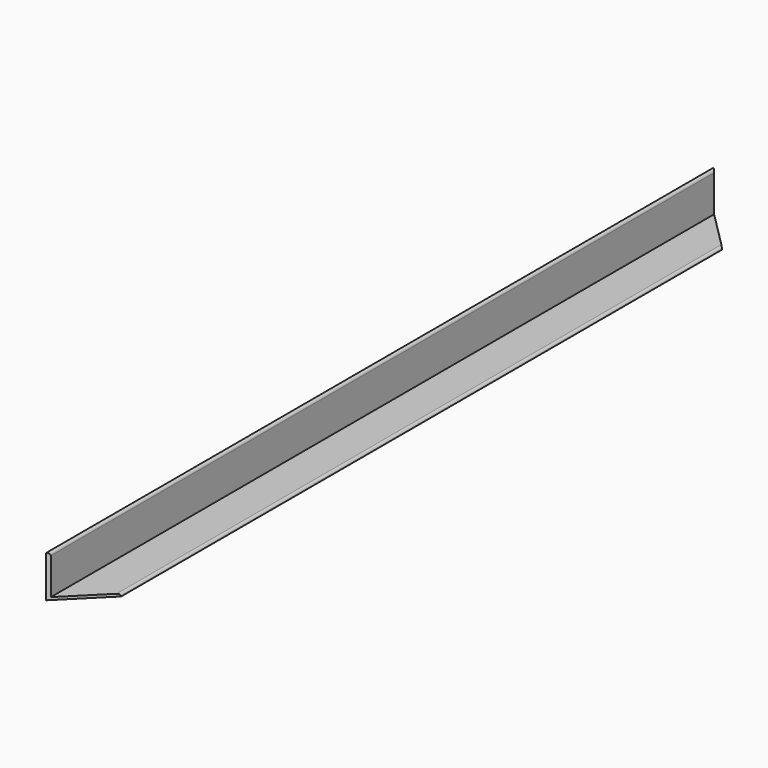
from build123d import *

# Parameters (mm, degrees)
F1_DEPTH = 508
F3_DEPTH = 50.8


# Not quite as in the source:
# - a pattern or mirror of a feature is missing from the dataset's text; its kind, count and spacing are read off the source's solid


with BuildPart() as f1:
    # F0 (on Front) → F1 (new body, symmetric)
    with BuildSketch(Plane.XZ):
        with BuildLine():
            ThreePointArc((-920.7500404358, 47.625), (-921.6799764055, 49.8700640303), (-923.9250404358, 50.8))
            Line((-923.9250404358, 50.8), (-923.9250404358, 0))
            Line((-923.9250404358, 0), (-873.1250404358, 0))
            ThreePointArc((-873.1250404358, 0), (-874.0549764055, 2.2450640303), (-876.3000404358, 3.175))
            Line((-876.3000404358, 3.175), (-920.7500404358, 3.175))
            Line((-920.7500404358, 3.175), (-920.7500404358, 47.625))
        make_face()
    extrude(amount=F1_DEPTH, both=True)

    # F2 (on face) → F3 (cut)
    with BuildSketch(Plane(origin=(0, 0, 0), x_dir=(1, 0, 0), z_dir=(0, 0, -1))):
        Polygon((-873.1250404358, -457.2), (-923.9250404358, -508), (-873.1250404358, -508), align=None)
    f3 = extrude(amount=-F3_DEPTH, mode=Mode.SUBTRACT)

    # F3_copies: F3 across plane
    add(f3.mirror(Plane(origin=(0, 0, 0), x_dir=(0, 0, -1), z_dir=(0, -1, 0))), mode=Mode.SUBTRACT)


solid = f1.part
